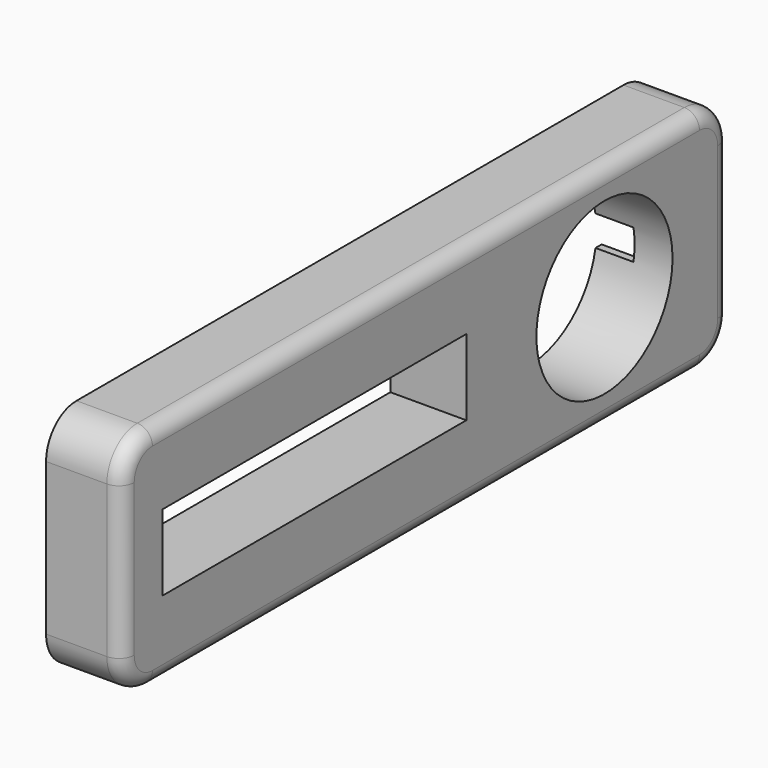
from build123d import *

# Parameters (mm, degrees)
F0_W     = 50
F0_H     = 10
F0_R     = 11.1985350655
F1_DEPTH = 10
F2_T     = -1
F3_R     = 2
F5_DEPTH = 5


with BuildPart() as f1:
    # F0 (on Right) → F1 (new body)
    with BuildSketch(Plane.YZ):
        with BuildLine():
            ThreePointArc((-50, -10), (-48.5355339059, -13.5355339059), (-45, -15))
            Line((-45, -15), (45, -15))
            ThreePointArc((45, -15), (48.5355339059, -13.5355339059), (50, -10))
            Line((50, -10), (50, 10))
            ThreePointArc((50, 10), (48.5355339059, 13.5355339059), (45, 15))
            Line((45, 15), (-45, 15))
            ThreePointArc((-45, 15), (-48.5355339059, 13.5355339059), (-50, 10))
            Line((-50, 10), (-50, -10))
        make_face()
        with Locations((-18.3541104198, 0)):
            Rectangle(F0_W, F0_H, mode=Mode.SUBTRACT)
        with Locations((29.37316522, 0)):
            Circle(F0_R, mode=Mode.SUBTRACT)
    extrude(amount=F1_DEPTH)

    # F2
    f2_openings = [f1.faces().sort_by_distance(p)[0] for p in [
        (0, -47.797293, 12.797293),
    ]]
    offset(amount=F2_T, openings=f2_openings, kind=Kind.INTERSECTION)

    # F3
    f3_edges = [f1.edges().sort_by_distance(p)[0] for p in [
        (10, 0, -15),
        (10, -48.535534, 13.535534),
        (10, -50, 0),
        (10, -48.535534, -13.535534),
        (10, 48.535534, -13.535534),
        (10, 50, 0),
        (10, 48.535534, 13.535534),
        (10, 0, 15),
    ]]
    fillet(f3_edges, radius=F3_R)

    # F4 (on face) → F5 (cut)
    with BuildSketch(Plane(origin=(0, 0, 0), x_dir=(0, -1, 0), z_dir=(-1, 0, 0))):
        with BuildLine():
            Line((-41.4066292992, 2), (-43.37316522, 2))
            Line((-43.37316522, 2), (-43.37316522, -2))
            Line((-43.37316522, -2), (-41.4066292992, -2))
            ThreePointArc((-41.4066292992, -2), (-41.5717002855, 0), (-41.4066292992, 2))
        make_face()
        with BuildLine():
            Line((-40.3916582029, 2), (-41.4066292992, 2))
            ThreePointArc((-41.4066292992, 2), (-41.5717002855, 0), (-41.4066292992, -2))
            Line((-41.4066292992, -2), (-40.3916582029, -2))
            ThreePointArc((-40.3916582029, -2), (-40.5717002855, 0), (-40.3916582029, 2))
        make_face()
        with BuildLine():
            Line((-18.3546722372, 2), (-40.3916582029, 2))
            ThreePointArc((-40.3916582029, 2), (-40.5717002855, 0), (-40.3916582029, -2))
            Line((-40.3916582029, -2), (-18.3546722372, -2))
            ThreePointArc((-18.3546722372, -2), (-18.2197314965, -1.0040437181), (-18.1746301545, 0))
            ThreePointArc((-18.1746301545, 0), (-18.2197314965, 1.0040437181), (-18.3546722372, 2))
        make_face()
        with BuildLine():
            ThreePointArc((-17.1746301545, 0), (-17.2159679428, 1.0034002729), (-17.3397011409, 2))
            Line((-17.3397011409, 2), (-18.3546722372, 2))
            ThreePointArc((-18.3546722372, 2), (-18.2197314965, 1.0040437181), (-18.1746301545, 0))
            ThreePointArc((-18.1746301545, 0), (-18.2197314965, -1.0040437181), (-18.3546722372, -2))
            Line((-18.3546722372, -2), (-17.3397011409, -2))
            ThreePointArc((-17.3397011409, -2), (-17.2159679428, -1.0034002729), (-17.1746301545, 0))
        make_face()
        with BuildLine():
            Line((-15.37316522, 2), (-17.3397011409, 2))
            ThreePointArc((-17.3397011409, 2), (-17.2159679428, 1.0034002729), (-17.1746301545, 0))
            ThreePointArc((-17.1746301545, 0), (-17.2159679428, -1.0034002729), (-17.3397011409, -2))
            Line((-17.3397011409, -2), (-15.37316522, -2))
            Line((-15.37316522, -2), (-15.37316522, 2))
        make_face()
    extrude(amount=-F5_DEPTH, mode=Mode.SUBTRACT)


solid = f1.part
